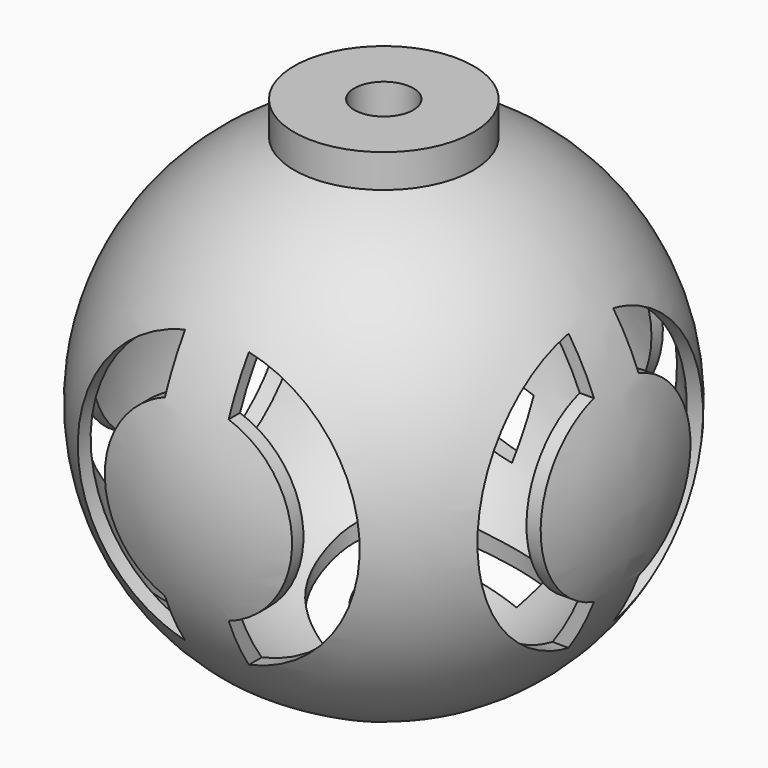
from build123d import *

# Parameters (mm, degrees)
F3_W          = 33.02
F3_H          = 33.02
F4_DEPTH      = 25.4
F5_T          = -2
F8_DEPTH      = 25.4
F9_DEPTH      = 25.4
F12_DEPTH     = 25.4
F15_DEPTH     = 25.4
F18_DEPTH     = 25.4
F20_TEXT_SIZE = 63.1530096547
F21_DEPTH     = 25.4
F22_R         = 13.6783186101
F22_R_2       = 6.2206430536
F22_R_3       = 4.4958
F23_DEPTH     = 5.08


# Not quite as in the source:
# - Text() gives the source's letters only with a copy of the font that has no kerning and outlines rounded to 1/6400 em; it was checked with that copy


with BuildPart() as f1:
    # F0 (on Front) → F1 (revolve)
    with BuildSketch(Plane.XZ):
        with BuildLine():
            Line((0, 38.1), (0, -38.1))
            ThreePointArc((0, -38.1), (38.1, 0), (0, 38.1))
        make_face()
    revolve(axis=Axis((0, 0, 0), (0, 0, 1)))

    # F3 (on offset) → F4 (cut)
    with BuildSketch(Plane.XY.offset(35.56)):
        Rectangle(F3_W, F3_H)
    extrude(amount=F4_DEPTH, mode=Mode.SUBTRACT)

    # F5
    f5_openings = [f1.faces().sort_by_distance(p)[0] for p in [
        (0, 0, 35.56),
    ]]
    offset(amount=F5_T, openings=f5_openings)

    # F7 (on offset) → F8 (cut)
    with BuildSketch(Plane.YZ.offset(38.1)):
        with BuildLine():
            Line((-4.1164528171, 13.6676668223), (-4.1164528171, 21.0943717888))
            ThreePointArc((-4.1164528171, 21.0943717888), (-21.4922708191, 0), (-4.1164528171, -21.0943717888))
            Line((-4.1164528171, -21.0943717888), (-4.1164528171, -13.6676668223))
            ThreePointArc((-4.1164528171, -13.6676668223), (-14.2741129378, 0), (-4.1164528171, 13.6676668223))
        make_face()
    extrude(amount=-F8_DEPTH, mode=Mode.SUBTRACT)

    # F7 (on offset) → F9 (cut)
    with BuildSketch(Plane.YZ.offset(38.1)):
        with BuildLine():
            Line((4.3820702894, 21.0407976308), (4.3820702894, 13.5848356685))
            ThreePointArc((4.3820702894, 13.5848356685), (14.2741129378, 0), (4.3820702894, -13.5848356685))
            Line((4.3820702894, -13.5848356685), (4.3820702894, -21.0407976308))
            ThreePointArc((4.3820702894, -21.0407976308), (21.4922708191, 0), (4.3820702894, 21.0407976308))
        make_face()
    extrude(amount=-F9_DEPTH, mode=Mode.SUBTRACT)

    # F11 (on offset) → F12 (cut)
    with BuildSketch(Plane.XZ.offset(-38.1)):
        with BuildLine():
            Line((-3.6698376409, 13.7950065868), (-3.6698376409, 21.1727094688))
            ThreePointArc((-3.6698376409, 21.1727094688), (-21.4884, 0), (-3.6698376409, -21.1727094688))
            Line((-3.6698376409, -21.1727094688), (-3.6698376409, -13.7950065868))
            ThreePointArc((-3.6698376409, -13.7950065868), (-14.2748, 0), (-3.6698376409, 13.7950065868))
        make_face()
        with BuildLine():
            Line((3.7780908185, -13.7657526059), (3.7780908185, -21.1536607784))
            ThreePointArc((3.7780908185, -21.1536607784), (21.4884, 0), (3.7780908185, 21.1536607784))
            Line((3.7780908185, 21.1536607784), (3.7780908185, 13.7657526059))
            ThreePointArc((3.7780908185, 13.7657526059), (14.2748, 0), (3.7780908185, -13.7657526059))
        make_face()
    extrude(amount=F12_DEPTH, mode=Mode.SUBTRACT)

    # F14 (on offset) → F15 (cut)
    with BuildSketch(Plane.YZ.offset(-38.1)):
        with BuildLine():
            ThreePointArc((-4.1349082105, -13.6628126362), (-14.2748, 0), (-4.1349082105, 13.6628126362))
            Line((-4.1349082105, 13.6628126362), (-4.1349082105, 21.086817414))
            ThreePointArc((-4.1349082105, 21.086817414), (-21.4884, 0), (-4.1349082105, -21.086817414))
            Line((-4.1349082105, -21.086817414), (-4.1349082105, -13.6628126362))
        make_face()
        with BuildLine():
            ThreePointArc((3.754181198, -21.1579171492), (21.4884, 0), (3.754181198, 21.1579171492))
            Line((3.754181198, 21.1579171492), (3.754181198, 13.7722924226))
            ThreePointArc((3.754181198, 13.7722924226), (14.2748, 0), (3.754181198, -13.7722924226))
            Line((3.754181198, -13.7722924226), (3.754181198, -21.1579171492))
        make_face()
    extrude(amount=F15_DEPTH, mode=Mode.SUBTRACT)

    # F17 (on offset) → F18 (cut)
    with BuildSketch(Plane.XZ.offset(38.1)):
        with BuildLine():
            ThreePointArc((-5.1061100354, -13.3303246527), (-14.2748, 0), (-5.1061100354, 13.3303246527))
            Line((-5.1061100354, 13.3303246527), (-5.1061100354, 20.8729244445))
            ThreePointArc((-5.1061100354, 20.8729244445), (-21.4884, 0), (-5.1061100354, -20.8729244445))
            Line((-5.1061100354, -20.8729244445), (-5.1061100354, -13.3303246527))
        make_face()
        with BuildLine():
            Line((4.5991366155, -13.5136174813), (4.5991366155, -20.9904568066))
            ThreePointArc((4.5991366155, -20.9904568066), (21.4884, 0), (4.5991366155, 20.9904568066))
            Line((4.5991366155, 20.9904568066), (4.5991366155, 13.5136174813))
            ThreePointArc((4.5991366155, 13.5136174813), (14.2748, 0), (4.5991366155, -13.5136174813))
        make_face()
    extrude(amount=-F18_DEPTH, mode=Mode.SUBTRACT)

    # F20 (on offset) → F21 (cut)
    with BuildSketch(Plane.XY.offset(-38.1)):
        with Locations((-21.2777052075, -22.8808205575)):
            Text('S', F20_TEXT_SIZE, font='Open Sans', text_align=(TextAlign.LEFT, TextAlign.BOTTOM))
    extrude(amount=F21_DEPTH, mode=Mode.SUBTRACT)

    # F22 (on face) → F23 (join)
    with BuildSketch(Plane.XY.offset(35.56)):
        Circle(F22_R)
        Circle(F22_R_2, mode=Mode.SUBTRACT)
        Circle(F22_R_2)
        Circle(F22_R_3, mode=Mode.SUBTRACT)
    extrude(amount=F23_DEPTH)


solid = f1.part
